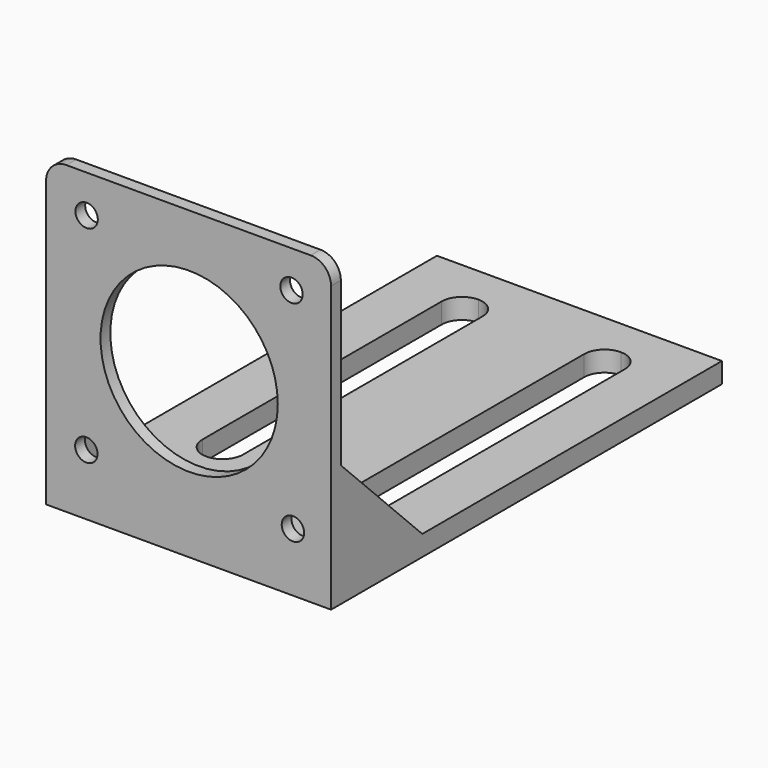
from build123d import *

# Parameters (mm, degrees)
F0_R      = 2.75
F1_DEPTH  = 3
F2_R      = 21.767
F3_DEPTH  = 25
F0_W      = 70
F0_H      = 5
F4_DEPTH  = 120
F6_DEPTH  = 25
F7_R      = 5
F9_DEPTH  = 3
F11_DEPTH = 3


# Not quite as in the source:
# - a feature names something its author has since deleted; it is built from what else it names


with BuildPart() as f1:
    # F0 (on Front) → F1 (new body)
    with BuildSketch(Plane.XZ):
        Polygon((-35.1443272789, 34.7749316851), (-35.1443272789, -30.2250683149), (-35.1443272789, -35.2250683149), (34.8556727211, -35.2250683149), (34.8556727211, 34.7749316851), align=None)
        Polygon((29.8556727211, -20.9088045945), (29.8556727211, -30.2250683149), (21.0454399179, -30.2250683149), (-20.0690244843, -30.2250683149), (-30.1443272789, -30.2250683149), (-30.1443272789, -20.0232621124), (-30.1443272789, 20.9646839807), (-30.1443272789, 29.7749316851), (-20.9545706917, 29.7749316851), (20.6652218889, 29.7749316851), (29.8556727211, 29.7749316851), (29.8556727211, 20.9646914313), align=None, mode=Mode.SUBTRACT)
        Polygon((-20.0690244843, -30.2250683149), (21.0454399179, -30.2250683149), (21.0454399179, -23.8184407195), (23.5755527805, -20.9088045945), (29.8556727211, -20.9088045945), (29.8556727211, 20.9646914313), (22.6900065731, 20.9646914313), (20.6652218889, 22.609265537), (20.6652218889, 29.7749316851), (-20.9545706917, 29.7749316851), (-20.9545706917, 23.6213151524), (-23.6111795117, 20.9646839807), (-30.1443272789, 20.9646839807), (-30.1443272789, -20.0232621124), (-22.8521441628, -20.0232621124), (-20.0690244843, -22.5533824255), align=None)
        Polygon((-30.1443272789, 29.7749316851), (-30.1443272789, 20.9646839807), (-23.6111795117, 20.9646839807), (-20.9545706917, 23.6213151524), (-20.9545706917, 29.7749316851), align=None)
        with Locations((-25.186798494, 25.5123097608)):
            Circle(F0_R, mode=Mode.SUBTRACT)
        Polygon((22.6900065731, 20.9646914313), (29.8556727211, 20.9646914313), (29.8556727211, 29.7749316851), (20.6652218889, 29.7749316851), (20.6652218889, 22.609265537), align=None)
        with Locations((25.1352448512, 25.6822819479)):
            Circle(F0_R, mode=Mode.SUBTRACT)
        Polygon((-30.1443272789, -30.2250683149), (-20.0690244843, -30.2250683149), (-20.0690244843, -22.5533824255), (-22.8521441628, -20.0232621124), (-30.1443272789, -20.0232621124), align=None)
        with Locations((-25.255761068, -25.2100098719)):
            Circle(F0_R, mode=Mode.SUBTRACT)
        Polygon((21.0454399179, -30.2250683149), (29.8556727211, -30.2250683149), (29.8556727211, -20.9088045945), (23.5755527805, -20.9088045945), (21.0454399179, -23.8184407195), align=None)
        with Locations((25.4847700376, -25.7638242348)):
            Circle(F0_R, mode=Mode.SUBTRACT)
    extrude(amount=-F1_DEPTH)

    # F2 (on face) → F3 (cut)
    with BuildSketch(Plane.XZ):
        Circle(F2_R)
    extrude(amount=-F3_DEPTH, mode=Mode.SUBTRACT)

    # F0 (on Front) → F4 (join)
    with BuildSketch(Plane.XZ):
        with Locations((-0.1443272789, -37.7250683149)):
            Rectangle(F0_W, F0_H)
    extrude(amount=-F4_DEPTH)

    # F5 (on face) → F6 (cut)
    with BuildSketch(Plane.XY.offset(-35.2250683149)):
        with BuildLine():
            Line((-17.5721636394, 90.75), (-12.5721636394, 90.75))
            ThreePointArc((-12.5721636394, 90.75), (-14.0366297335, 94.2855339059), (-17.5721636394, 95.75))
            Line((-17.5721636394, 95.75), (-17.5721636394, 90.75))
        make_face()
        with BuildLine():
            ThreePointArc((-17.5721636394, 95.75), (-21.1076975454, 94.2855339059), (-22.5721636394, 90.75))
            Line((-22.5721636394, 90.75), (-17.5721636394, 90.75))
            Line((-17.5721636394, 90.75), (-17.5721636394, 95.75))
        make_face()
        with BuildLine():
            Line((-17.5721636394, 90.75), (-22.5721636394, 90.75))
            ThreePointArc((-22.5721636394, 90.75), (-21.1076975454, 87.2144660941), (-17.5721636394, 85.75))
            Line((-17.5721636394, 85.75), (-17.5721636394, 90.75))
        make_face()
        with BuildLine():
            ThreePointArc((-17.5721636394, 85.75), (-14.0366297335, 87.2144660941), (-12.5721636394, 90.75))
            Line((-12.5721636394, 90.75), (-17.5721636394, 90.75))
            Line((-17.5721636394, 90.75), (-17.5721636394, 85.75))
        make_face()
        with BuildLine():
            Line((-12.5721636394, 32.25), (-12.5721636394, 90.75))
            ThreePointArc((-12.5721636394, 90.75), (-14.0366297335, 87.2144660941), (-17.5721636394, 85.75))
            Line((-17.5721636394, 85.75), (-17.5721636394, 37.25))
            ThreePointArc((-17.5721636394, 37.25), (-14.0366297335, 35.7855339059), (-12.5721636394, 32.25))
        make_face()
        with BuildLine():
            ThreePointArc((-17.5721636394, 85.75), (-21.1076975454, 87.2144660941), (-22.5721636394, 90.75))
            Line((-22.5721636394, 90.75), (-22.5721636394, 32.25))
            ThreePointArc((-22.5721636394, 32.25), (-21.1076975454, 35.7855339059), (-17.5721636394, 37.25))
            Line((-17.5721636394, 37.25), (-17.5721636394, 85.75))
        make_face()
        with BuildLine():
            ThreePointArc((-17.5721636394, 37.25), (-21.1076975454, 35.7855339059), (-22.5721636394, 32.25))
            Line((-22.5721636394, 32.25), (-17.5721636394, 32.25))
            Line((-17.5721636394, 32.25), (-17.5721636394, 37.25))
        make_face()
        with BuildLine():
            Line((-17.5721636394, 32.25), (-12.5721636394, 32.25))
            ThreePointArc((-12.5721636394, 32.25), (-14.0366297335, 35.7855339059), (-17.5721636394, 37.25))
            Line((-17.5721636394, 37.25), (-17.5721636394, 32.25))
        make_face()
        with BuildLine():
            ThreePointArc((-17.5721636394, 27.25), (-14.0366297335, 28.7144660941), (-12.5721636394, 32.25))
            Line((-12.5721636394, 32.25), (-17.5721636394, 32.25))
            Line((-17.5721636394, 32.25), (-17.5721636394, 27.25))
        make_face()
        with BuildLine():
            Line((-17.5721636394, 32.25), (-22.5721636394, 32.25))
            ThreePointArc((-22.5721636394, 32.25), (-21.1076975454, 28.7144660941), (-17.5721636394, 27.25))
            Line((-17.5721636394, 27.25), (-17.5721636394, 32.25))
        make_face()
        with BuildLine():
            Line((22.4278363606, 32.25), (22.4278363606, 90.75))
            ThreePointArc((22.4278363606, 90.75), (20.9633702665, 87.2144660941), (17.4278363606, 85.75))
            Line((17.4278363606, 85.75), (17.4278363606, 37.25))
            ThreePointArc((17.4278363606, 37.25), (20.9633702665, 35.7855339059), (22.4278363606, 32.25))
        make_face()
        with BuildLine():
            Line((17.4278363606, 90.75), (12.4278363606, 90.75))
            ThreePointArc((12.4278363606, 90.75), (13.8923024546, 87.2144660941), (17.4278363606, 85.75))
            Line((17.4278363606, 85.75), (17.4278363606, 90.75))
        make_face()
        with BuildLine():
            ThreePointArc((17.4278363606, 95.75), (13.8923024546, 94.2855339059), (12.4278363606, 90.75))
            Line((12.4278363606, 90.75), (17.4278363606, 90.75))
            Line((17.4278363606, 90.75), (17.4278363606, 95.75))
        make_face()
        with BuildLine():
            Line((17.4278363606, 90.75), (22.4278363606, 90.75))
            ThreePointArc((22.4278363606, 90.75), (20.9633702665, 94.2855339059), (17.4278363606, 95.75))
            Line((17.4278363606, 95.75), (17.4278363606, 90.75))
        make_face()
        with BuildLine():
            ThreePointArc((17.4278363606, 85.75), (20.9633702665, 87.2144660941), (22.4278363606, 90.75))
            Line((22.4278363606, 90.75), (17.4278363606, 90.75))
            Line((17.4278363606, 90.75), (17.4278363606, 85.75))
        make_face()
        with BuildLine():
            ThreePointArc((17.4278363606, 85.75), (13.8923024546, 87.2144660941), (12.4278363606, 90.75))
            Line((12.4278363606, 90.75), (12.4278363606, 32.25))
            ThreePointArc((12.4278363606, 32.25), (13.8923024546, 35.7855339059), (17.4278363606, 37.25))
            Line((17.4278363606, 37.25), (17.4278363606, 85.75))
        make_face()
        with BuildLine():
            ThreePointArc((17.4278363606, 37.25), (13.8923024546, 35.7855339059), (12.4278363606, 32.25))
            Line((12.4278363606, 32.25), (17.4278363606, 32.25))
            Line((17.4278363606, 32.25), (17.4278363606, 37.25))
        make_face()
        with BuildLine():
            Line((17.4278363606, 32.25), (22.4278363606, 32.25))
            ThreePointArc((22.4278363606, 32.25), (20.9633702665, 35.7855339059), (17.4278363606, 37.25))
            Line((17.4278363606, 37.25), (17.4278363606, 32.25))
        make_face()
        with BuildLine():
            ThreePointArc((17.4278363606, 27.25), (20.9633702665, 28.7144660941), (22.4278363606, 32.25))
            Line((22.4278363606, 32.25), (17.4278363606, 32.25))
            Line((17.4278363606, 32.25), (17.4278363606, 27.25))
        make_face()
        with BuildLine():
            Line((17.4278363606, 32.25), (12.4278363606, 32.25))
            ThreePointArc((12.4278363606, 32.25), (13.8923024546, 28.7144660941), (17.4278363606, 27.25))
            Line((17.4278363606, 27.25), (17.4278363606, 32.25))
        make_face()
        with BuildLine():
            ThreePointArc((-17.5721636394, 100.75), (-21.1076975454, 102.2144660941), (-22.5721636394, 105.75))
            Line((-22.5721636394, 105.75), (-22.5721636394, 90.75))
            ThreePointArc((-22.5721636394, 90.75), (-21.1076975454, 94.2855339059), (-17.5721636394, 95.75))
            Line((-17.5721636394, 95.75), (-17.5721636394, 100.75))
        make_face()
        with BuildLine():
            Line((-12.5721636394, 90.75), (-12.5721636394, 105.75))
            ThreePointArc((-12.5721636394, 105.75), (-14.0366297335, 102.2144660941), (-17.5721636394, 100.75))
            Line((-17.5721636394, 100.75), (-17.5721636394, 95.75))
            ThreePointArc((-17.5721636394, 95.75), (-14.0366297335, 94.2855339059), (-12.5721636394, 90.75))
        make_face()
        with BuildLine():
            ThreePointArc((17.4278363606, 100.75), (13.8923024546, 102.2144660941), (12.4278363606, 105.75))
            Line((12.4278363606, 105.75), (12.4278363606, 90.75))
            ThreePointArc((12.4278363606, 90.75), (13.8923024546, 94.2855339059), (17.4278363606, 95.75))
            Line((17.4278363606, 95.75), (17.4278363606, 100.75))
        make_face()
        with BuildLine():
            Line((22.4278363606, 90.75), (22.4278363606, 105.75))
            ThreePointArc((22.4278363606, 105.75), (20.9633702665, 102.2144660941), (17.4278363606, 100.75))
            Line((17.4278363606, 100.75), (17.4278363606, 95.75))
            ThreePointArc((17.4278363606, 95.75), (20.9633702665, 94.2855339059), (22.4278363606, 90.75))
        make_face()
        with BuildLine():
            Line((22.4278363606, 105.75), (17.4278363606, 105.75))
            Line((17.4278363606, 105.75), (17.4278363606, 100.75))
            ThreePointArc((17.4278363606, 100.75), (20.9633702665, 102.2144660941), (22.4278363606, 105.75))
        make_face()
        with BuildLine():
            ThreePointArc((22.4278363606, 105.75), (20.9633702665, 109.2855339059), (17.4278363606, 110.75))
            Line((17.4278363606, 110.75), (17.4278363606, 105.75))
            Line((17.4278363606, 105.75), (22.4278363606, 105.75))
        make_face()
        with BuildLine():
            Line((17.4278363606, 105.75), (17.4278363606, 110.75))
            ThreePointArc((17.4278363606, 110.75), (13.8923024546, 109.2855339059), (12.4278363606, 105.75))
            Line((12.4278363606, 105.75), (17.4278363606, 105.75))
        make_face()
        with BuildLine():
            Line((-17.5721636394, 105.75), (-17.5721636394, 110.75))
            ThreePointArc((-17.5721636394, 110.75), (-21.1076975454, 109.2855339059), (-22.5721636394, 105.75))
            Line((-22.5721636394, 105.75), (-17.5721636394, 105.75))
        make_face()
        with BuildLine():
            ThreePointArc((-12.5721636394, 105.75), (-14.0366297335, 109.2855339059), (-17.5721636394, 110.75))
            Line((-17.5721636394, 110.75), (-17.5721636394, 105.75))
            Line((-17.5721636394, 105.75), (-12.5721636394, 105.75))
        make_face()
        with BuildLine():
            Line((-12.5721636394, 105.75), (-17.5721636394, 105.75))
            Line((-17.5721636394, 105.75), (-17.5721636394, 100.75))
            ThreePointArc((-17.5721636394, 100.75), (-14.0366297335, 102.2144660941), (-12.5721636394, 105.75))
        make_face()
        with BuildLine():
            Line((-17.5721636394, 105.75), (-22.5721636394, 105.75))
            ThreePointArc((-22.5721636394, 105.75), (-21.1076975454, 102.2144660941), (-17.5721636394, 100.75))
            Line((-17.5721636394, 100.75), (-17.5721636394, 105.75))
        make_face()
        with BuildLine():
            Line((17.4278363606, 105.75), (12.4278363606, 105.75))
            ThreePointArc((12.4278363606, 105.75), (13.8923024546, 102.2144660941), (17.4278363606, 100.75))
            Line((17.4278363606, 100.75), (17.4278363606, 105.75))
        make_face()
    extrude(amount=-F6_DEPTH, mode=Mode.SUBTRACT)

    # F7
    f7_edges = [f1.edges().sort_by_distance(p)[0] for p in [
        (-35.144327, 1.5, 34.774932),
        (34.855673, 1.5, 34.774932),
    ]]
    fillet(f7_edges, radius=F7_R)

    # F8 (on face) → F9 (join)
    with BuildSketch(Plane(origin=(-35.1443272789, 0, 0), x_dir=(0, -1, 0), z_dir=(-1, 0, 0))):
        Polygon((-28, -35.2250683149), (-3, -35.2250683149), (-3, -10.2250683149), align=None)
    extrude(amount=-F9_DEPTH)

    # F10 (on face) → F11 (join)
    with BuildSketch(Plane.YZ.offset(34.8556727211)):
        Polygon((3, -10.2250683149), (3, -35.2250683149), (28, -35.2250683149), align=None)
    extrude(amount=-F11_DEPTH)


solid = f1.part
